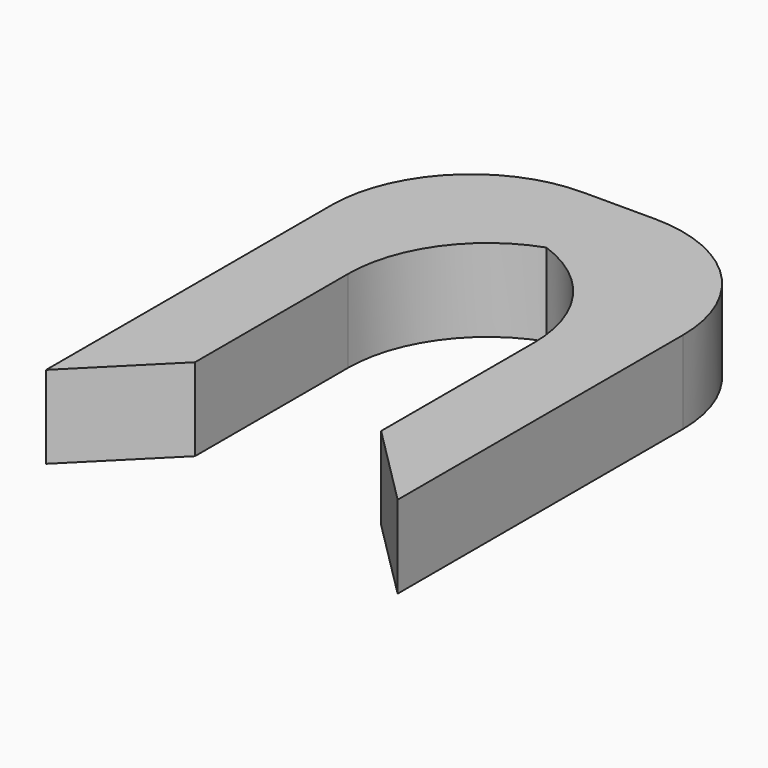
from build123d import *

# Parameters (mm, degrees)
F0_W        = 4.5
F0_H        = 2
F1_DEPTH    = 2
F2_T1_DEPTH = 2
F2_T3_DEPTH = 18.8994949366
F3_SIZE     = 1.99999


# Not quite as in the source:
# - a fillet or chamfer that OpenCascade refuses, or shapes differently, is made with other operations: its cross-section is extruded or revolved along the edge and cut away or added
# - a fillet or chamfer is up to 0.001 mm smaller than in the source, because OpenCascade refuses the exact size


with BuildPart() as f1:
    # F0 (on Top) → F1 (new body)
    with BuildSketch(Plane.XY):
        Polygon((0, 12), (0, 0), (2, 0), (2, 10), (2, 12), align=None)
        Polygon((6.5, 12), (6.5, 10), (6.5, 0), (8.5, 0), (8.5, 12), align=None)
        with Locations((4.25, 11)):
            Rectangle(F0_W, F0_H)
    extrude(amount=F1_DEPTH)

    # F2: fillet of radius 3.3798989873 on 4 edges, made by hand

    # F2_s2 → F2_t1 (join)
    with BuildSketch(Plane.XY):
        with BuildLine():
            ThreePointArc((3.1201010127, 10), (5.5100505063, 9.0100505063), (6.5, 6.6201010127))
            Line((6.5, 6.6201010127), (6.5, 10))
            Line((6.5, 10), (3.1201010127, 10))
        make_face()
        with BuildLine():
            ThreePointArc((2, 6.6201010127), (2.9899494937, 9.0100505063), (5.3798989873, 10))
            Line((5.3798989873, 10), (2, 10))
            Line((2, 10), (2, 6.6201010127))
        make_face()
    extrude(amount=F2_T1_DEPTH)

    # F2_s4 → F2_t3 (cut)
    with BuildSketch(Plane.XY.offset(-8.4497474683)):
        with BuildLine():
            ThreePointArc((0, 8.6201010127), (0.9899494937, 11.0100505063), (3.3798989873, 12))
            Line((3.3798989873, 12), (0, 12))
            Line((0, 12), (0, 8.6201010127))
        make_face()
        with BuildLine():
            ThreePointArc((5.1201010127, 12), (7.5100505063, 11.0100505063), (8.5, 8.6201010127))
            Line((8.5, 8.6201010127), (8.5, 12))
            Line((8.5, 12), (5.1201010127, 12))
        make_face()
    extrude(amount=F2_T3_DEPTH, mode=Mode.SUBTRACT)

    # F3 (size 2 in the source; OpenCascade refuses exactly that, so slightly less here)
    f3_edges = [f1.edges().sort_by_distance(p)[0] for p in [
        (2, 0, 1),
        (6.5, 0, 1),
    ]]
    chamfer(f3_edges, length=F3_SIZE)


solid = f1.part
